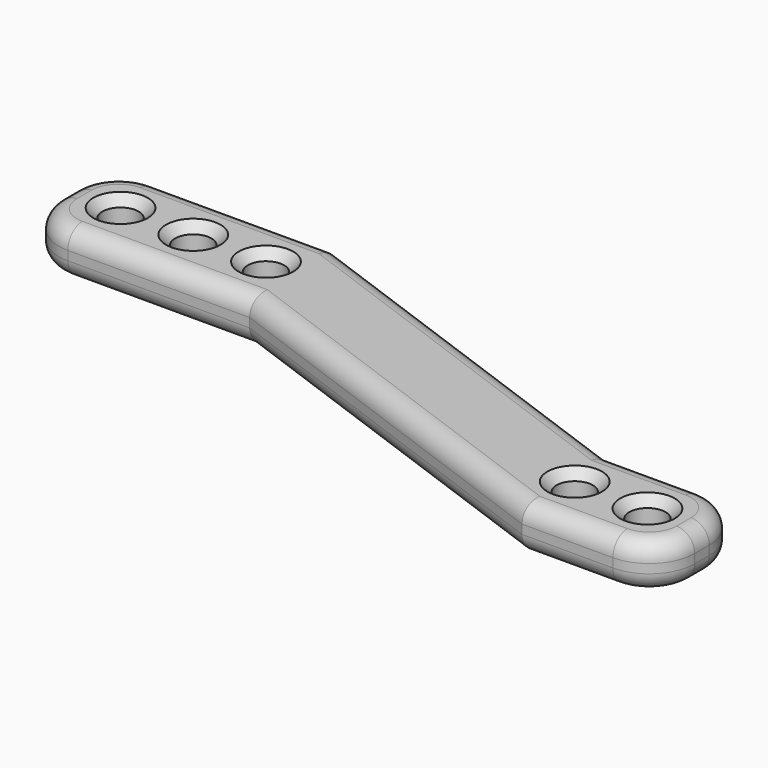
from build123d import *

# Parameters (mm, degrees)
F0_W         = 25
F0_H         = 12
F0_W_2       = 15
F1_DEPTH     = 5
F2_R         = 2
F3_DEPTH     = 5.001
F4_R         = 2
F5_T1_DEPTH  = 5
F5_T4_ANGLE  = 90
F5_T6_ANGLE  = 90
F5_T8_ANGLE  = 90
F5_T10_ANGLE = 90
F5_T12_ANGLE = 90
F5_T14_ANGLE = 90
F5_T16_ANGLE = 90
F5_T18_ANGLE = 90
F6_SIZE      = 1


# Not quite as in the source:
# - a fillet or chamfer that OpenCascade refuses, or shapes differently, is made with other operations: its cross-section is extruded or revolved along the edge and cut away or added


with BuildPart() as f1:
    # F0 (on Top) → F1 (new body)
    with BuildSketch(Plane.XY):
        with Locations((-12.5, -6)):
            Rectangle(F0_W, F0_H)
        Polygon((42.2861679354, -15.3909064497), (0, 0), (0, -12), (42.2861679354, -27.3909064497), align=None)
        with Locations((49.7861679354, -21.3909064497)):
            Rectangle(F0_W_2, F0_H)
    extrude(amount=F1_DEPTH)

    # F2 (on Top) → F3 (cut, through all)
    with BuildSketch(Plane.XY):
        with Locations((51.2861679354, -21.3909064497)):
            Circle(F2_R)
        with Locations((-19, -6)):
            Circle(F2_R)
        with Locations((43.2861679354, -21.3909064497)):
            Circle(F2_R)
        with Locations((-11, -6)):
            Circle(F2_R)
        with Locations((-3, -6)):
            Circle(F2_R)
    extrude(amount=F3_DEPTH, mode=Mode.SUBTRACT)

    # F4
    f4_edges = [f1.edges().sort_by_distance(p)[0] for p in [
        (21.143084, -19.695453, 5),
        (21.143084, -7.695453, 5),
        (-12.5, -12, 5),
        (-12.5, 0, 5),
        (49.786168, -27.390906, 5),
        (57.286168, -21.390906, 5),
        (49.786168, -15.390906, 5),
        (49.786168, -27.390906, 0),
        (21.143084, -19.695453, 0),
        (-12.5, -12, 0),
        (57.286168, -21.390906, 0),
        (21.143084, -7.695453, 0),
        (49.786168, -15.390906, 0),
        (-12.5, 0, 0),
        (-25, -6, 0),
        (-25, -6, 5),
    ]]
    fillet(f4_edges, radius=F4_R)

    # F5: fillet of radius 5 on 4 edges, made by hand

    # F5_s2 → F5_t1 (cut)
    with BuildSketch(Plane.XY):
        with BuildLine():
            ThreePointArc((52.2861679354, -15.3909064497), (55.8217018413, -16.8553725437), (57.2861679354, -20.3909064497))
            Line((57.2861679354, -20.3909064497), (57.2861679354, -15.3909064497))
            Line((57.2861679354, -15.3909064497), (52.2861679354, -15.3909064497))
        make_face()
        with BuildLine():
            ThreePointArc((-20, 0), (-23.5355339059, -1.4644660941), (-25, -5))
            Line((-25, -5), (-25, 0))
            Line((-25, 0), (-20, 0))
        make_face()
        with BuildLine():
            ThreePointArc((-25, -7), (-23.5355339059, -10.5355339059), (-20, -12))
            Line((-20, -12), (-25, -12))
            Line((-25, -12), (-25, -7))
        make_face()
        with BuildLine():
            ThreePointArc((57.2861679354, -22.3909064497), (55.8217018413, -25.9264403556), (52.2861679354, -27.3909064497))
            Line((52.2861679354, -27.3909064497), (57.2861679354, -27.3909064497))
            Line((57.2861679354, -27.3909064497), (57.2861679354, -22.3909064497))
        make_face()
    extrude(amount=F5_T1_DEPTH, mode=Mode.SUBTRACT)

    # F5_s3 → F5_t4 (revolve, cut)
    with BuildSketch(Plane.YZ.offset(52.2861679354)):
        with BuildLine():
            ThreePointArc((-25.3909064497, 5), (-26.805120012, 4.4142135624), (-27.3909064497, 3))
            Line((-27.3909064497, 3), (-27.3909064497, 5))
            Line((-27.3909064497, 5), (-25.3909064497, 5))
        make_face()
    revolve(axis=Axis((52.2861679354, -22.3909064497, 5), (0, 0, 1)), revolution_arc=F5_T4_ANGLE, mode=Mode.SUBTRACT)

    # F5_s5 → F5_t6 (revolve, cut)
    with BuildSketch(Plane.XZ.offset(7)):
        with BuildLine():
            ThreePointArc((-23, 5), (-24.4142135624, 4.4142135624), (-25, 3))
            Line((-25, 3), (-25, 5))
            Line((-25, 5), (-23, 5))
        make_face()
    revolve(axis=Axis((-20, -7, 5), (0, 0, 1)), revolution_arc=F5_T6_ANGLE, mode=Mode.SUBTRACT)

    # F5_s7 → F5_t8 (revolve, cut)
    with BuildSketch(Plane.YZ.offset(-20)):
        with BuildLine():
            ThreePointArc((-2, 5), (-0.5857864376, 4.4142135624), (0, 3))
            Line((0, 3), (0, 5))
            Line((0, 5), (-2, 5))
        make_face()
    revolve(axis=Axis((-20, -5, 5), (0, 0, 1)), revolution_arc=F5_T8_ANGLE, mode=Mode.SUBTRACT)

    # F5_s9 → F5_t10 (revolve, cut)
    with BuildSketch(Plane.XZ.offset(5)):
        with BuildLine():
            ThreePointArc((-23, 0), (-24.4142135624, 0.5857864376), (-25, 2))
            Line((-25, 2), (-25, 0))
            Line((-25, 0), (-23, 0))
        make_face()
    revolve(axis=Axis((-20, -5, 0), (0, 0, -1)), revolution_arc=F5_T10_ANGLE, mode=Mode.SUBTRACT)

    # F5_s11 → F5_t12 (revolve, cut)
    with BuildSketch(Plane.YZ.offset(-20)):
        with BuildLine():
            ThreePointArc((-10, 0), (-11.4142135624, 0.5857864376), (-12, 2))
            Line((-12, 2), (-12, 0))
            Line((-12, 0), (-10, 0))
        make_face()
    revolve(axis=Axis((-20, -7, 0), (0, 0, -1)), revolution_arc=F5_T12_ANGLE, mode=Mode.SUBTRACT)

    # F5_s13 → F5_t14 (revolve, cut)
    with BuildSketch(Plane.XZ.offset(22.3909064497)):
        with BuildLine():
            ThreePointArc((55.2861679354, 0), (56.7003814977, 0.5857864376), (57.2861679354, 2))
            Line((57.2861679354, 2), (57.2861679354, 0))
            Line((57.2861679354, 0), (55.2861679354, 0))
        make_face()
    revolve(axis=Axis((52.2861679354, -22.3909064497, 0), (0, 0, -1)), revolution_arc=F5_T14_ANGLE, mode=Mode.SUBTRACT)

    # F5_s15 → F5_t16 (revolve, cut)
    with BuildSketch(Plane.YZ.offset(52.2861679354)):
        with BuildLine():
            ThreePointArc((-17.3909064497, 0), (-15.9766928873, 0.5857864376), (-15.3909064497, 2))
            Line((-15.3909064497, 2), (-15.3909064497, 0))
            Line((-15.3909064497, 0), (-17.3909064497, 0))
        make_face()
    revolve(axis=Axis((52.2861679354, -20.3909064497, 0), (0, 0, -1)), revolution_arc=F5_T16_ANGLE, mode=Mode.SUBTRACT)

    # F5_s17 → F5_t18 (revolve, cut)
    with BuildSketch(Plane.XZ.offset(20.3909064497)):
        with BuildLine():
            ThreePointArc((55.2861679354, 5), (56.7003814977, 4.4142135624), (57.2861679354, 3))
            Line((57.2861679354, 3), (57.2861679354, 5))
            Line((57.2861679354, 5), (55.2861679354, 5))
        make_face()
    revolve(axis=Axis((52.2861679354, -20.3909064497, 5), (0, 0, 1)), revolution_arc=F5_T18_ANGLE, mode=Mode.SUBTRACT)

    # F6
    f6_edges = [f1.edges().sort_by_distance(p)[0] for p in [
        (-21, -6, 5),
        (-13, -6, 5),
        (-5, -6, 5),
        (41.286168, -21.390906, 5),
        (49.286168, -21.390906, 5),
    ]]
    chamfer(f6_edges, length=F6_SIZE)


solid = f1.part
